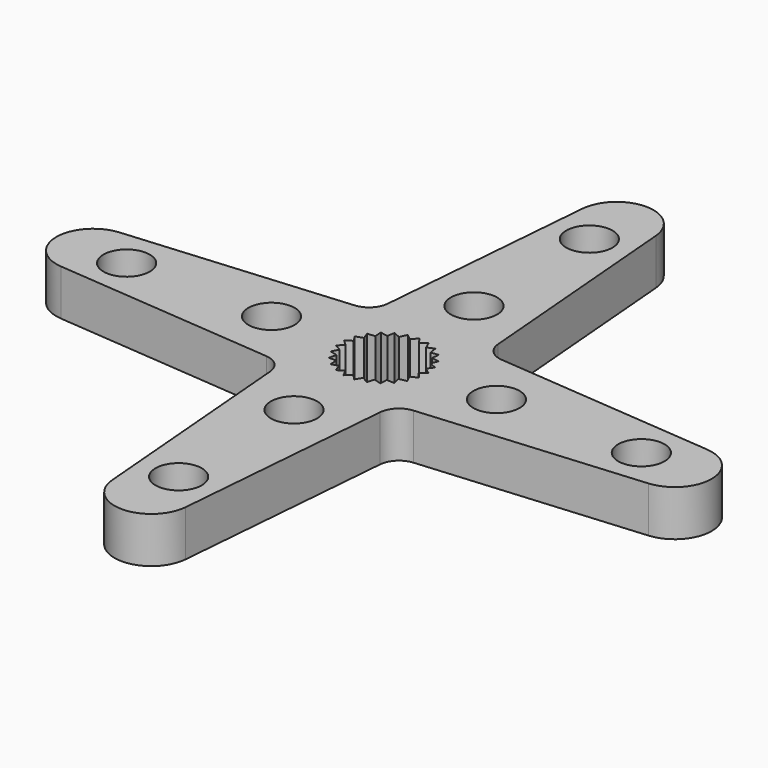
from build123d import *

# Parameters (mm, degrees)
F0_R     = 1.6
F1_DEPTH = 3.175


# Not quite as in the source:
# - a length typed as a fraction of an inch, garbled in the dataset ("3 / 203.2 mm" for 3/8 in), is restored


with BuildPart() as f1:
    # F0 (on Top) → F1 (new body)
    with BuildSketch(Plane.XY):
        with BuildLine():
            ThreePointArc((-3.8043671626, 5.08), (-4.2086486587, 4.2104292787), (-5.08, 3.81))
            Line((-5.08, 3.81), (-20.32, 2.54))
            ThreePointArc((-20.32, 2.54), (-22.6579985335, 0), (-20.32, -2.54))
            Line((-20.32, -2.54), (-5.08, -3.8043671626))
            ThreePointArc((-5.08, -3.8043671626), (-4.2121628624, -4.2103745873), (-3.81, -5.08))
            Line((-3.81, -5.08), (-2.54, -20.32))
            ThreePointArc((-2.54, -20.32), (0, -22.6579985335), (2.54, -20.32))
            Line((2.54, -20.32), (3.8043671626, -5.08))
            ThreePointArc((3.8043671626, -5.08), (4.2103745873, -4.2121628624), (5.08, -3.81))
            Line((5.08, -3.81), (20.32, -2.54))
            ThreePointArc((20.32, -2.54), (22.6579985335, 0), (20.32, 2.54))
            Line((20.32, 2.54), (5.08, 3.8043671626))
            ThreePointArc((5.08, 3.8043671626), (4.2121628624, 4.2103745873), (3.81, 5.08))
            Line((3.81, 5.08), (2.54, 20.32))
            ThreePointArc((2.54, 20.32), (0, 22.6579985335), (-2.54, 20.32))
            Line((-2.54, 20.32), (-3.8043671626, 5.08))
        make_face()
        with Locations((-17.7799620532, -0.0219527348)):
            Circle(F0_R, mode=Mode.SUBTRACT)
        with Locations((-7.7799861494, 0)):
            Circle(F0_R, mode=Mode.SUBTRACT)
        with Locations((0.0219527348, -17.7799620532)):
            Circle(F0_R, mode=Mode.SUBTRACT)
        with Locations((0, -7.7799861494)):
            Circle(F0_R, mode=Mode.SUBTRACT)
        with Locations((7.7799861494, 0)):
            Circle(F0_R, mode=Mode.SUBTRACT)
        with Locations((-0.0219527348, 17.7799620532)):
            Circle(F0_R, mode=Mode.SUBTRACT)
        Polygon((-2.3131272616, 1.150841372), (-2.4811892868, 1.651717782), (-1.9542535042, 1.6899369317), (-1.992472654, 2.2168727143), (-1.4725868119, 2.1228475389), (-1.3785616365, 2.6427333809), (-0.8983920744, 2.4223718279), (-0.6780305213, 2.90254139), (-0.2677480588, 2.5696895861), (0.0651037451, 2.9799720486), (0.379719552, 2.555544297), (0.8041473037, 2.8701601039), (1.0033279869, 2.380824761), (1.4926633298, 2.5800054442), (1.5638936344, 2.0565092492), (2.0873898293, 2.1277395538), (2.0261940932, 1.6029756981), (2.5509579489, 1.5417799619), (2.3611813253, 1.0487212884), (2.8542399989, 0.8589446648), (2.547806851, 0.4285718633), (2.9781796525, 0.1221387154), (2.574344302, -0.2185063082), (2.9149893256, -0.6223416587), (2.4391262327, -0.8518549247), (2.6686394987, -1.3277180175), (2.1506488918, -1.4316783634), (2.2546092377, -1.9496689703), (1.7270383715, -1.9215441851), (1.6989135863, -2.4491150513), (1.1949116786, -2.2906723188), (1.0364689461, -2.7946742265), (0.5877042905, -2.5158690862), (0.3088991502, -2.9646337418), (-0.0564307197, -2.5829845462), (-0.4380799154, -2.9483144161), (-0.6970199802, -2.4878015876), (-1.1575328087, -2.7467416524), (-1.2938129119, -2.2363009057), (-1.8042536586, -2.3725810089), (-1.80931082, -1.8442852134), (-2.3376066155, -1.8493423749), (-2.2111230752, -1.3363862984), (-2.7240791517, -1.209902758), (-2.4740023355, -0.7445173173), (-2.9393877762, -0.4944405012), (-2.5814309304, -0.105867575), (-2.9700038565, 0.2520892708), (-2.5266587261, 0.5394342163), (-2.8140036716, 0.9827793468), align=None, mode=Mode.SUBTRACT)
        with Locations((0, 7.7799861494)):
            Circle(F0_R, mode=Mode.SUBTRACT)
        with Locations((17.7799620532, 0.0219527348)):
            Circle(F0_R, mode=Mode.SUBTRACT)
    extrude(amount=F1_DEPTH)


solid = f1.part
